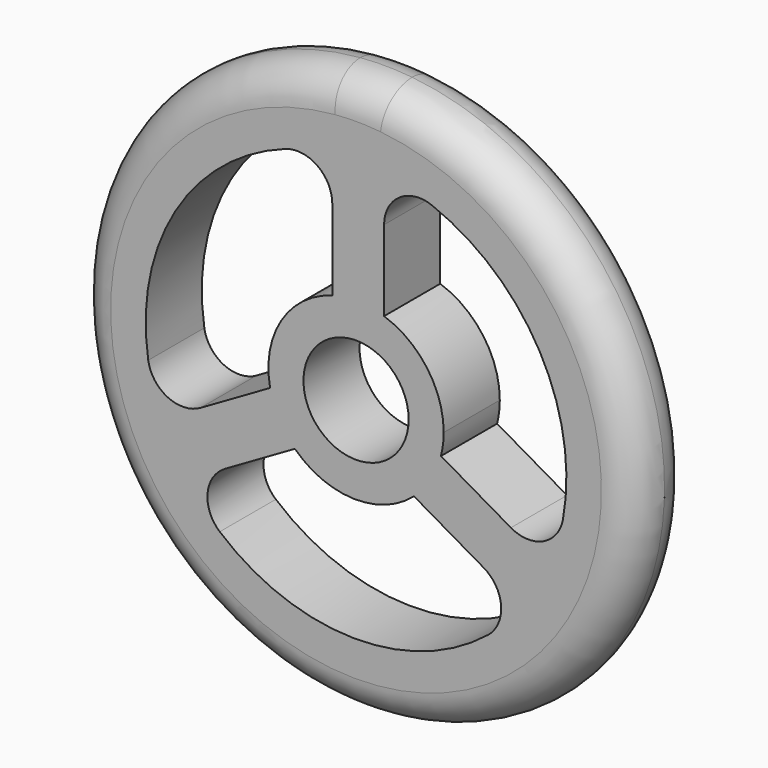
from build123d import *

# Parameters (mm, degrees)
F0_R     = 7.5
F1_DEPTH = 10
F2_R     = 4.99999


# Not quite as in the source:
# - a fillet or chamfer is up to 0.001 mm smaller than in the source, because OpenCascade refuses the exact size


with BuildPart() as f1:
    # F0 (on Front) → F1 (new body)
    with BuildSketch(Plane.XZ):
        with BuildLine():
            ThreePointArc((-3.3902032697, 39.8560725836), (-27.0591192504, -29.4585143107), (40, 0))
            ThreePointArc((40, 0), (29.6647939484, 26.83281573), (4, 39.7994974843))
            ThreePointArc((4, 39.7994974843), (0.3062077702, 39.9988279428), (-3.3902032697, 39.8560725836))
        make_face()
        with BuildLine():
            ThreePointArc((-29.6388118521, -4.6412101868), (-25.7834406394, 15.3366941937), (-10.0682439236, 28.2600506775))
            ThreePointArc((-10.0682439236, 28.2600506775), (-5.5083812132, 27.6360062099), (-3.3902032697, 23.5500422312))
            Line((-3.3902032697, 23.5500422312), (-3.3902032697, 12.0314804488))
            ThreePointArc((-3.3902032697, 12.0314804488), (0.3191719091, 12.4959245073), (4, 11.8427192823))
            Line((4, 11.8427192823), (4, 23.3238075794))
            ThreePointArc((4, 23.3238075794), (6.1715728753, 27.446913205), (10.8, 27.9885690953))
            ThreePointArc((10.8, 27.9885690953), (26.1736871016, 14.6607674939), (29.5080437608, -5.4106703294))
            ThreePointArc((29.5080437608, -5.4106703294), (26.6876740435, -9.0476050406), (22.0900364673, -8.8390189601))
            Line((22.0900364673, -8.8390189601), (12.1146693487, -3.0797380689))
            ThreePointArc((12.1146693487, -3.0797380689), (10.6622021125, -6.5243732351), (8.2560957484, -9.3854612563))
            Line((8.2560957484, -9.3854612563), (18.1990098767, -15.1260054048))
            ThreePointArc((18.1990098767, -15.1260054048), (20.6839376534, -19.0681954938), (18.8388118521, -23.3473589085))
            ThreePointArc((18.8388118521, -23.3473589085), (-0.3902464621, -29.9974616876), (-19.4397998371, -22.8493803481))
            ThreePointArc((-19.4397998371, -22.8493803481), (-21.1792928303, -18.5884011693), (-18.6998331976, -14.7110232712))
            Line((-18.6998331976, -14.7110232712), (-8.724466079, -8.95174238))
            ThreePointArc((-8.724466079, -8.95174238), (-10.9813740217, -5.9715512722), (-12.2560957484, -2.457258026))
            Line((-12.2560957484, -2.457258026), (-22.1990098767, -8.1978021746))
            ThreePointArc((-22.1990098767, -8.1978021746), (-26.8555105286, -8.3787177112), (-29.6388118521, -4.6412101868))
        make_face(mode=Mode.SUBTRACT)
        with BuildLine():
            ThreePointArc((4, 11.8427192823), (0.3191719091, 12.4959245073), (-3.3902032697, 12.0314804488))
            ThreePointArc((-3.3902032697, 12.0314804488), (-10.6622021125, 6.5243732351), (-12.2560957484, -2.457258026))
            ThreePointArc((-12.2560957484, -2.457258026), (-10.9813740217, -5.9715512722), (-8.724466079, -8.95174238))
            ThreePointArc((-8.724466079, -8.95174238), (-0.3191719091, -12.4959245073), (8.2560957484, -9.3854612563))
            ThreePointArc((8.2560957484, -9.3854612563), (10.6622021125, -6.5243732351), (12.1146693487, -3.0797380689))
            ThreePointArc((12.1146693487, -3.0797380689), (12.4032932493, -1.5518751789), (12.5, 0))
            ThreePointArc((12.5, 0), (10.1550480058, 7.2886898686), (4, 11.8427192823))
        make_face()
        Circle(F0_R, mode=Mode.SUBTRACT)
    extrude(amount=F1_DEPTH)

    # F2 (radius 5 in the source; OpenCascade refuses exactly that, so slightly less here)
    f2_edges = [f1.edges().sort_by_distance(p)[0] for p in [
        (-40, -10, 0),
        (-40, 0, 0),
    ]]
    fillet(f2_edges, radius=F2_R)


solid = f1.part
